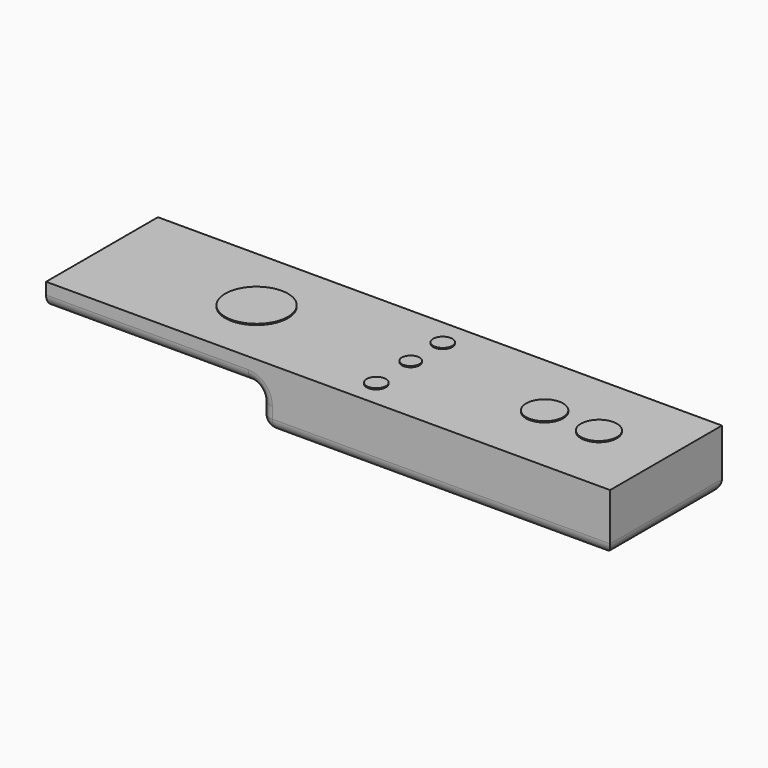
from build123d import *

# Parameters (mm, degrees)
F0_W        = 237.3272180557
F0_H        = 58.8164292276
F1_DEPTH    = 10
F2_W        = 147.2023129463
F2_H        = 58.8164292276
F3_DEPTH    = 15
F4_F1_R     = 5.08
F4_F2_R     = 5.08
F5_W        = 55.2143082023
F5_H        = 22.0865048468
F6_DEPTH    = 4
F7_T1_DEPTH = 46.9058521388
F7_T3_DEPTH = 80.0336554942
F9_R        = 13.2118644906
F10_DEPTH   = 0.5
F11_R       = 4.0488978151
F12_DEPTH   = 0.5
F11_R_2     = 3.7300649458
F11_R_3     = 4.0152102199
F11_R_4     = 7.8029945449
F11_R_5     = 7.5839402098


# Not quite as in the source:
# - a fillet or chamfer that OpenCascade refuses, or shapes differently, is made with other operations: its cross-section is extruded or revolved along the edge and cut away or added


with BuildPart() as f1:
    # F0 (on Top) → F1 (new body)
    with BuildSketch(Plane.XY):
        Rectangle(F0_W, F0_H)
    extrude(amount=F1_DEPTH)

    # F2 (on face) → F3 (join)
    with BuildSketch(Plane(origin=(0, 0, 0), x_dir=(1, 0, 0), z_dir=(0, 0, -1))):
        with Locations((45.0624525547, 0)):
            Rectangle(F2_W, F2_H)
    extrude(amount=F3_DEPTH)

    # F4: fillet of radius 5.08 on 7 edges, made by hand

    # F4_f1
    f4_f1_edges = [f1.edges().sort_by_distance(p)[0] for p in [
        (-28.5387039185, 0, 0),
    ]]
    fillet(f4_f1_edges, radius=F4_F1_R)

    # F4_f2
    f4_f2_edges = [f1.edges().sort_by_distance(p)[0] for p in [
        (-28.5387039185, -29.4082146138, -10.04),
        (-28.5387039185, 29.4082146138, -10.04),
        (-28.5387039185, 0, -15),
        (45.0624525547, 29.4082146138, -15),
        (118.6636090279, 0, -15),
        (45.0624525547, -29.4082146138, -15),
        (-30.02660147, 29.4082146138, -1.4878975516),
        (-30.02660147, -29.4082146138, -1.4878975516),
    ]]
    fillet(f4_f2_edges, radius=F4_F2_R)

    # F5 (on face) → F6 (join)
    with BuildSketch(Plane(origin=(0, 0, 0), x_dir=(1, 0, 0), z_dir=(0, 0, -1))):
        with Locations((-83.400927484, 0)):
            Rectangle(F5_W, F5_H)
    extrude(amount=F6_DEPTH)

    # F7: fillet of radius 5.08 on 4 edges, made by hand

    # F7_s2 → F7_t1 (cut)
    with BuildSketch(Plane.XZ.offset(-23.4529260694)):
        with BuildLine():
            ThreePointArc((-55.7937733829, 0), (-57.5701673512, -2.8755530587), (-60.7576428413, -4))
            Line((-60.7576428413, -4), (-55.7937733829, -4))
            Line((-55.7937733829, -4), (-55.7937733829, 0))
        make_face()
        with BuildLine():
            ThreePointArc((-111.0080815852, 0), (-109.2316876169, -2.8755530587), (-106.0442121268, -4))
            Line((-106.0442121268, -4), (-111.0080815852, -4))
            Line((-111.0080815852, -4), (-111.0080815852, 0))
        make_face()
    extrude(amount=F7_T1_DEPTH, mode=Mode.SUBTRACT)

    # F7_s4 → F7_t3 (cut)
    with BuildSketch(Plane.YZ.offset(-123.4177552312)):
        with BuildLine():
            ThreePointArc((-11.0432524234, 0), (-9.2668584551, -2.8755530587), (-6.079382965, -4))
            Line((-6.079382965, -4), (-11.0432524234, -4))
            Line((-11.0432524234, -4), (-11.0432524234, 0))
        make_face()
        with BuildLine():
            ThreePointArc((11.0432524234, 0), (9.2668584551, -2.8755530587), (6.079382965, -4))
            Line((6.079382965, -4), (11.0432524234, -4))
            Line((11.0432524234, -4), (11.0432524234, 0))
        make_face()
    extrude(amount=F7_T3_DEPTH, mode=Mode.SUBTRACT)

    # F9 (on face) → F10 (join)
    with BuildSketch(Plane.XY.offset(10)):
        with Locations((-53.6077320576, 0)):
            Circle(F9_R)
    extrude(amount=F10_DEPTH)


with BuildPart() as f12:
    # F11 (on face) → F12 (new body)
    with BuildSketch(Plane.XY.offset(10.5)):
        with Locations((12.0495855808, -19.1157609224)):
            Circle(F11_R)
    extrude(amount=F12_DEPTH)


with BuildPart() as f12b:
    # F11 (on face) → F12, piece 2 (new body)
    with BuildSketch(Plane.XY.offset(10.5)):
        with Locations((11.2095503137, 0)):
            Circle(F11_R_2)
    extrude(amount=F12_DEPTH)


with BuildPart() as f12c:
    # F11 (on face) → F12, piece 3 (new body)
    with BuildSketch(Plane.XY.offset(10.5)):
        with Locations((11.2095503137, 16.8793648481)):
            Circle(F11_R_3)
    extrude(amount=F12_DEPTH)


with BuildPart() as f12d:
    # F11 (on face) → F12, piece 4 (new body)
    with BuildSketch(Plane.XY.offset(10.5)):
        with Locations((67.5813481212, 0)):
            Circle(F11_R_4)
    extrude(amount=F12_DEPTH)


with BuildPart() as f12e:
    # F11 (on face) → F12, piece 5 (new body)
    with BuildSketch(Plane.XY.offset(10.5)):
        with Locations((90.4404297471, 0)):
            Circle(F11_R_5)
    extrude(amount=F12_DEPTH)


solid = Compound([f1.part, f12.part, f12b.part, f12c.part, f12d.part, f12e.part])
